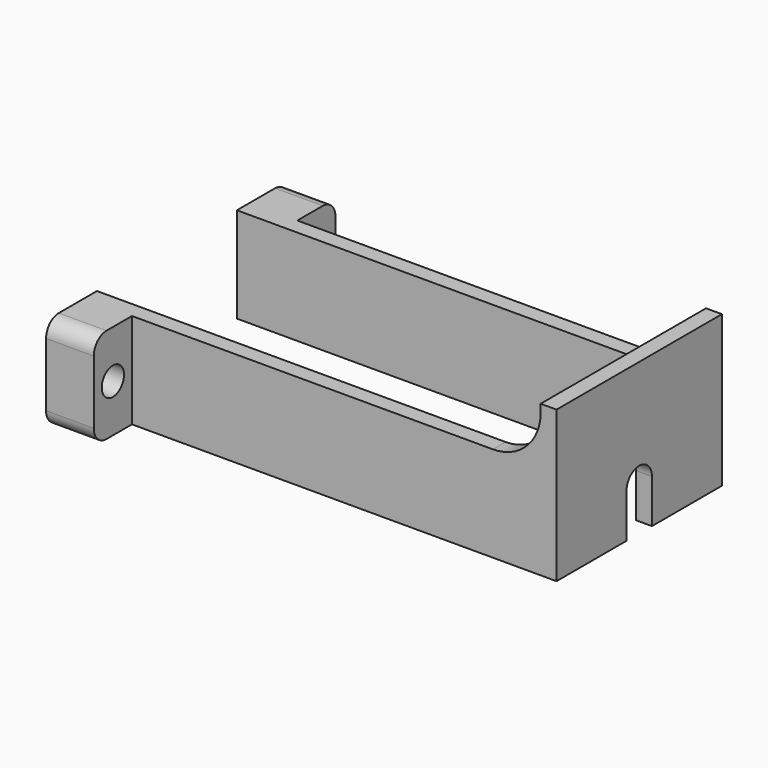
from build123d import *

# Parameters (mm, degrees)
F1_DEPTH  = 12
F3_DEPTH  = 4
F2_R      = 1.75
F4_DEPTH  = 25
F5_R      = 2
F8_DEPTH  = 25
F9_W      = 2
F9_H      = 26
F10_DEPTH = 7
F11_R     = 6
F12_R     = 1.99999


# Not quite as in the source:
# - a fillet or chamfer is up to 0.001 mm smaller than in the source, because OpenCascade refuses the exact size


with BuildPart() as f1:
    # F0 (on Top) → F1 (new body)
    with BuildSketch(Plane.XY):
        Polygon((2, 15.0915228184), (0, 15.0915228184), (0, 7.0915228184), (57.4, 7.0915228184), (57.4, -3.9084771816), (59.4, -3.9084771816), (59.4, 9.0915228184), (2, 9.0915228184), align=None)
    extrude(amount=F1_DEPTH)

    # F3 (add): a face of the model
    f3_faces = [f1.faces().sort_by_distance(p)[0] for p in [
        (2, 12.0915228184, 6),
    ]]
    extrude(f3_faces, amount=F3_DEPTH)

    # F2 (on face) → F4 (cut)
    with BuildSketch(Plane(origin=(0, 0, 0), x_dir=(0, -1, 0), z_dir=(-1, 0, 0))):
        with Locations((-12.0915228184, 6)):
            Circle(F2_R)
    extrude(amount=-F4_DEPTH, mode=Mode.SUBTRACT)

    # F5
    f5_edges = [f1.edges().sort_by_distance(p)[0] for p in [
        (3, 15.091523, 0),
        (3, 15.091523, 12),
    ]]
    fillet(f5_edges, radius=F5_R)

    # F6: F1 across face


with BuildPart() as f1_1:
    add(f1.part)
    add(f1.part.mirror(Plane(origin=(58.4, -3.9084771816, 6), x_dir=(1, 0, 0), z_dir=(0, -1, 0))))

    # F7 (on face) → F8 (cut)
    with BuildSketch(Plane.YZ.offset(59.4)):
        Polygon((-1.9084771816, 7.5), (-3.9084771816, 7.5), (-5.9084771816, 7.5), (-5.9084771816, 0), (-1.9084771816, 0), align=None)
    extrude(amount=-F8_DEPTH, mode=Mode.SUBTRACT)

    # F9 (on face) → F10 (join)
    with BuildSketch(Plane.XY.offset(12)):
        with Locations((58.4, -3.9084771816)):
            Rectangle(F9_W, F9_H)
    extrude(amount=F10_DEPTH)

    # F11
    f11_edges = [f1_1.edges().sort_by_distance(p)[0] for p in [
        (57.4, -15.908477, 12),
        (57.4, 8.091523, 12),
    ]]
    fillet(f11_edges, radius=F11_R)

    # F12 (radius 2 in the source; OpenCascade refuses exactly that, so slightly less here)
    f12_edges = [f1_1.edges().sort_by_distance(p)[0] for p in [
        (58.4, -1.908477, 7.5),
        (58.4, -5.908477, 7.5),
    ]]
    fillet(f12_edges, radius=F12_R)


solid = f1_1.part
